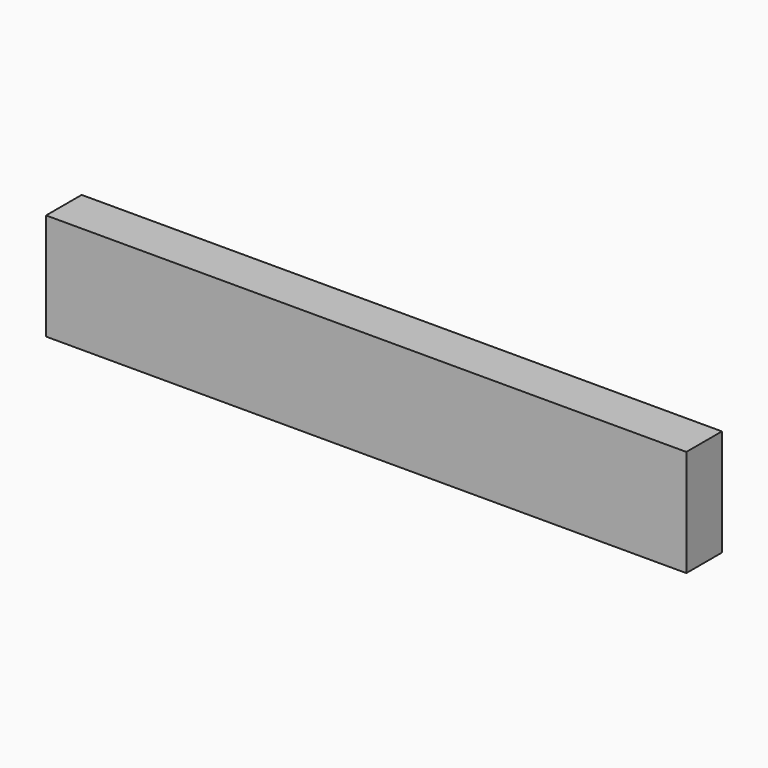
from build123d import *

# Parameters (mm, degrees)
F0_W     = 45.72
F0_H     = 7.62
F1_DEPTH = 3.175


# Not quite as in the source:
# - the program builds the solid bodies; features that only make, move or delete a surface that nothing else refers to are left out


with BuildPart() as f1:
    # F0 (on Front) → F1 (new body)
    with BuildSketch(Plane.XZ):
        with Locations((22.86, 3.81)):
            Rectangle(F0_W, F0_H)
    extrude(amount=F1_DEPTH)


solid = f1.part
